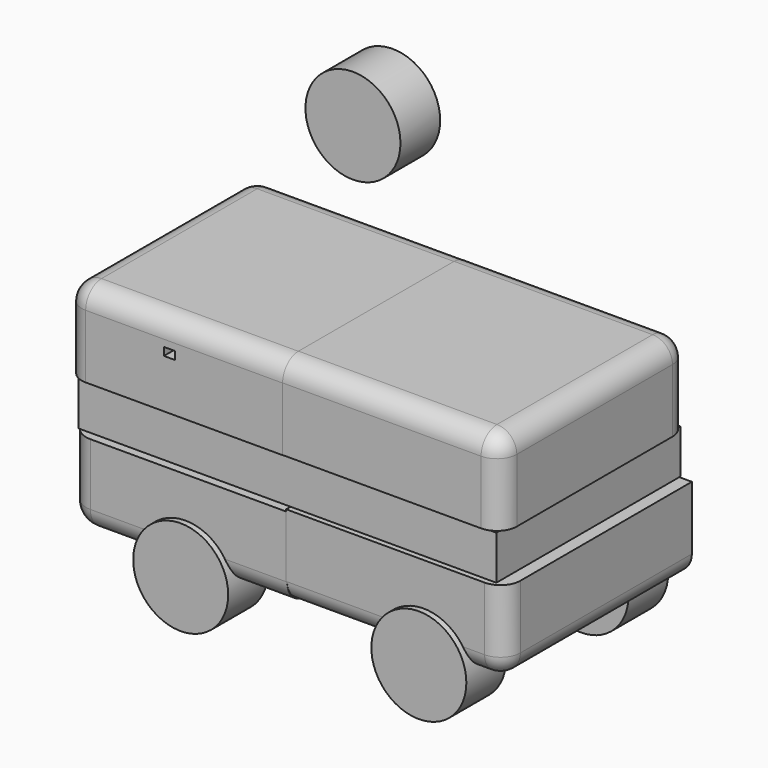
from build123d import *

# Parameters (mm, degrees)
F0_W         = 107.0024116431
F0_H         = 11.2637076527
F1_DEPTH     = 58.928
F2_W         = 55.88
F2_H         = 21.336
F2_W_2       = 2.8315708041
F2_H_2       = 2.0329207182
F3_DEPTH     = 59.944
F6_R         = 5.08
F7_T1_DEPTH  = 67.564
F7_S5_W      = 5.08
F7_S5_H      = 5.08
F7_T6_DEPTH  = 5.08
F8_R         = 5.08
F15_R        = 5.08
F16_T1_DEPTH = 63.5
F16_S5_W     = 5.08
F16_S5_H     = 5.08
F16_T6_DEPTH = 5.08
F17_R        = 5.5188922036
F18_R        = 12.1594429824
F19_DEPTH    = 12.7
F22_R        = 5.08
F22_2_R      = 5.08


# Not quite as in the source:
# - a fillet or chamfer that OpenCascade refuses, or shapes differently, is made with other operations: its cross-section is extruded or revolved along the edge and cut away or added


with BuildPart() as f1:
    # F0 (on Front) → F1 (new body)
    with BuildSketch(Plane.XZ):
        Rectangle(F0_W, F0_H)
    extrude(amount=F1_DEPTH)


with BuildPart() as f3:
    # F2 (on Front) → F3 (new body)
    with BuildSketch(Plane.XZ):
        with Locations((-27.94, 32.1588905327)):
            Rectangle(F2_W, F2_H)
        with Locations((-29.3557854021, 34.9952988327)):
            Rectangle(F2_W_2, F2_H_2, mode=Mode.SUBTRACT)
    extrude(amount=F3_DEPTH)


with BuildPart() as f3b:
    # F2 (on Front) → F3, piece 2 (new body)
    with BuildSketch(Plane.XZ):
        with Locations((42.02524625, 32.4493067138)):
            Rectangle(F2_W, F2_H)
    extrude(amount=F3_DEPTH)

    # F8
    f8_edges = [f3b.edges().sort_by_distance(p)[0] for p in [
        (42.025246, -59.944, 43.117307),
        (69.965246, -29.972, 43.117307),
        (69.965246, -59.944, 32.449307),
    ]]
    fillet(f8_edges, radius=F8_R)


with BuildPart() as f3c:
    # F2 (on Front) → F3, piece 3 (new body)
    with BuildSketch(Plane.XZ):
        with Locations((-27.94, -26.2150114603)):
            Rectangle(F2_W, F2_H)
    extrude(amount=F3_DEPTH)


with BuildPart() as f3d:
    # F2 (on Front) → F3, piece 4 (new body)
    with BuildSketch(Plane.XZ):
        with Locations((43.186915631, -26.2150114603)):
            Rectangle(F2_W, F2_H)
    extrude(amount=F3_DEPTH)


with BuildPart() as f4_1:
    # F4: copy of F3
    add(f3.part.moved(Location((0, 0, -15.494))))

    # F6
    f6_edges = [f4_1.edges().sort_by_distance(p)[0] for p in [
        (-55.88, -59.944, 16.664891),
        (-27.94, -59.944, 27.332891),
    ]]
    fillet(f6_edges, radius=F6_R)

    # F7: fillet of radius 5.08 on 1 edges, made by hand

    # F7_s2 → F7_t1 (cut)
    with BuildSketch(Plane.XZ.offset(-12.7)):
        with BuildLine():
            ThreePointArc((-50.8, 27.3328905327), (-54.3921024484, 25.8449929812), (-55.88, 22.2528905327))
            Line((-55.88, 22.2528905327), (-55.88, 27.3328905327))
            Line((-55.88, 27.3328905327), (-50.8, 27.3328905327))
        make_face()
    extrude(amount=F7_T1_DEPTH, mode=Mode.SUBTRACT)


with BuildPart() as f7_tool4:
    # F7_s5 → F7_t6 (new body)
    with BuildSketch(Plane.XY.offset(22.2528905327)):
        with Locations((-53.34, -57.404)):
            Rectangle(F7_S5_W, F7_S5_H)
    extrude(amount=F7_T6_DEPTH)

    # F7_s7 → F7_t8 (revolve, cut)
    with BuildSketch(Plane(origin=(-50.8, -54.864, 22.2528905327), x_dir=(0.7071067812, 0.7071067812, 0), z_dir=(0.7071067812, -0.7071067812, 0))):
        with BuildLine():
            ThreePointArc((0, -5.08), (5.08, 0), (0, 5.08))
            Line((0, 5.08), (0, -5.08))
        make_face()
    revolve(axis=Axis((-50.8, -54.864, 22.2528905327), (0, 0, 1)), mode=Mode.SUBTRACT)


with BuildPart() as f4_1_1:
    add(f4_1.part)

    # F7_t3: cut F7_tool4
    add(f7_tool4.part, mode=Mode.SUBTRACT)

    # F22
    f22_edges = [f4_1_1.edges().sort_by_distance(p)[0] for p in [
        (-55.88, 0, 14.124891),
    ]]
    fillet(f22_edges, radius=F22_R)


with BuildPart() as f9_1:
    # F9: copy of F3b
    add(f3b.part.moved(Location((-14.478, 0, -15.748))))

    # F22#2
    f22_2_edges = [f9_1.edges().sort_by_distance(p)[0] for p in [
        (55.487246, 0, 14.161307),
    ]]
    fillet(f22_2_edges, radius=F22_2_R)


with BuildPart() as f11_1:
    # F11: copy of F3c
    add(f3c.part.moved(Location((0.762, 0, 9.144))))

    # F17
    f17_edges = [f11_1.edges().sort_by_distance(p)[0] for p in [
        (-27.178, -59.944, -27.739011),
        (-55.118, -59.944, -17.071011),
        (-55.118, -29.972, -27.739011),
    ]]
    fillet(f17_edges, radius=F17_R)


with BuildPart() as f13_1:
    # F13: copy of F3d
    add(f3d.part.moved(Location((-14.732, 0, 9.652))))

    # F15
    f15_edges = [f13_1.edges().sort_by_distance(p)[0] for p in [
        (56.394916, -29.972, -27.231011),
        (56.394916, -59.944, -16.563011),
    ]]
    fillet(f15_edges, radius=F15_R)

    # F16: fillet of radius 5.08 on 1 edges, made by hand

    # F16_s2 → F16_t1 (cut)
    with BuildSketch(Plane.YZ.offset(-12.185084369)):
        with BuildLine():
            ThreePointArc((-59.944, -22.1510114603), (-58.4561024484, -25.7431139087), (-54.864, -27.2310114603))
            Line((-54.864, -27.2310114603), (-59.944, -27.2310114603))
            Line((-59.944, -27.2310114603), (-59.944, -22.1510114603))
        make_face()
    extrude(amount=F16_T1_DEPTH, mode=Mode.SUBTRACT)


with BuildPart() as f16_tool4:
    # F16_s5 → F16_t6 (new body)
    with BuildSketch(Plane.XZ.offset(54.864)):
        with Locations((53.854915631, -24.6910114603)):
            Rectangle(F16_S5_W, F16_S5_H)
    extrude(amount=F16_T6_DEPTH)

    # F16_s7 → F16_t8 (revolve, cut)
    with BuildSketch(Plane(origin=(51.314915631, -54.864, -22.1510114603), x_dir=(-0.7071067812, 0, 0.7071067812), z_dir=(0.7071067812, 0, 0.7071067812))):
        with BuildLine():
            ThreePointArc((0, -5.08), (5.08, 0), (0, 5.08))
            Line((0, 5.08), (0, -5.08))
        make_face()
    revolve(axis=Axis((51.314915631, -54.864, -22.1510114603), (0, -1, 0)), mode=Mode.SUBTRACT)


with BuildPart() as f13_1_1:
    add(f13_1.part)

    # F16_t3: cut F16_tool4
    add(f16_tool4.part, mode=Mode.SUBTRACT)


with BuildPart() as f19:
    # F18 (on Front) → F19 (new body)
    with BuildSketch(Plane.XZ):
        with Locations((-20.1840121299, 54.5984767377)):
            Circle(F18_R)
    extrude(amount=F19_DEPTH)


with BuildPart() as f20_1:
    # F20: copy of F19
    add(f19.part.moved(Location((-5.08, -48.768, -83.566))))


with BuildPart() as f21_1:
    # F21: copy of F19
    add(f19.part.moved(Location((55.88, -48.768, -83.566))))


with BuildPart() as f23_1:
    # F23: copy of F19
    add(f19.part.moved(Location((-4.826, 0, -83.312))))


with BuildPart() as f24_1:
    # F24: copy of F19
    add(f19.part.moved(Location((57.15, 1.524, -84.074))))


solid = Compound([f1.part, f4_1_1.part, f9_1.part, f11_1.part, f13_1_1.part, f19.part, f20_1.part, f21_1.part, f23_1.part, f24_1.part])
